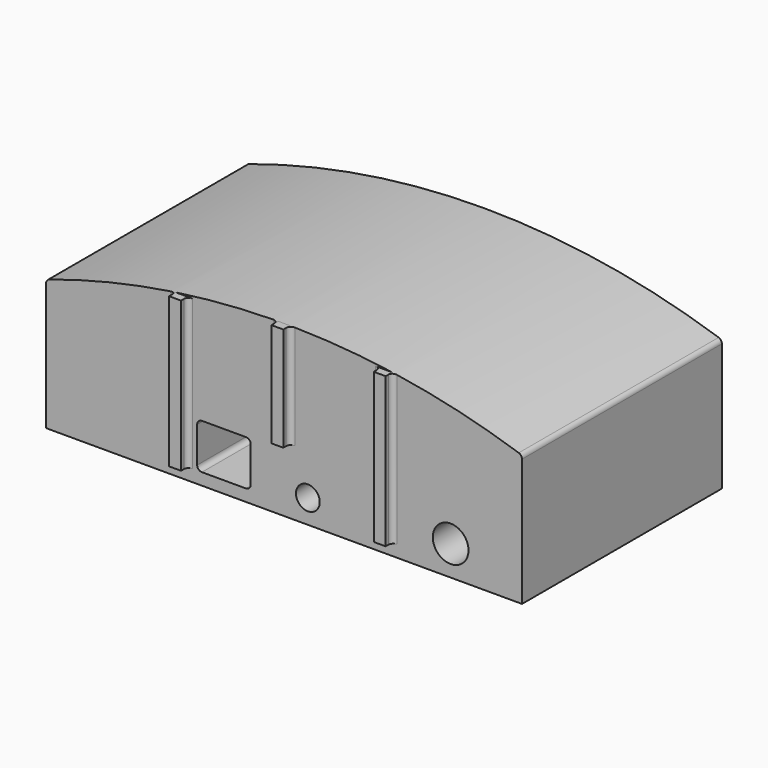
from build123d import *

# Parameters (mm, degrees)
F0_W         = 450
F0_H         = 380
F0_R         = 100
F0_R_2       = 150
F1_DEPTH     = 1050
F2_W         = 100
F2_H         = 1259.1041287501
F2_H_2       = 874.8020976761
F3_DEPTH     = 70
F4_T1_DEPTH  = 2100
F4_T3_DEPTH  = 1259.1041287501
F4_T8_DEPTH  = 1259.1041287501
F4_S9_R      = 6316.3461538462
F4_T10_DEPTH = 632
F4_T14_DEPTH = 874.8020976761
F4_S15_R     = 6316.3461538462
F4_T16_DEPTH = 440
F4_T20_DEPTH = 874.8020976761
F4_S21_R     = 6316.3461538462
F4_T22_DEPTH = 440
F4_T26_DEPTH = 1259.1041287501
F4_S27_R     = 6316.3461538462
F4_T28_DEPTH = 632
F4_T29_DEPTH = 2244.8937294243


# Not quite as in the source:
# - a fillet or chamfer that OpenCascade refuses, or shapes differently, is made with other operations: its cross-section is extruded or revolved along the edge and cut away or added


with BuildPart() as f1:
    # F0 (on Front) → F1 (new body, symmetric)
    with BuildSketch(Plane.XZ):
        with BuildLine():
            Line((-2000, -550), (2000, -550))
            Line((2000, -550), (2000, 550))
            ThreePointArc((2000, 550), (0, 875), (-2000, 550))
            Line((-2000, 550), (-2000, -550))
        make_face()
        with Locations((-505, -260)):
            Rectangle(F0_W, F0_H, mode=Mode.SUBTRACT)
        with Locations((200, -350)):
            Circle(F0_R, mode=Mode.SUBTRACT)
        with Locations((1400, -300)):
            Circle(F0_R_2, mode=Mode.SUBTRACT)
    extrude(amount=F1_DEPTH, both=True)

    # F2 (on face) → F3 (join)
    with BuildSketch(Plane.XZ.offset(1050)):
        with Locations((-860, 179.552064375)):
            Rectangle(F2_W, F2_H)
        with Locations((0, 437.401048838)):
            Rectangle(F2_W, F2_H_2)
        with Locations((860, 179.552064375)):
            Rectangle(F2_W, F2_H)
    extrude(amount=F3_DEPTH)

    # F4: fillet of radius 40 on 12 edges, made by hand

    # F4_s2 → F4_t1 (join)
    with BuildSketch(Plane.XZ.offset(-1050)):
        with BuildLine():
            ThreePointArc((-730, -410), (-718.2842712475, -438.2842712475), (-690, -450))
            Line((-690, -450), (-730, -450))
            Line((-730, -450), (-730, -410))
        make_face()
        with BuildLine():
            ThreePointArc((-730, -110), (-718.2842712475, -81.7157287525), (-690, -70))
            Line((-690, -70), (-730, -70))
            Line((-730, -70), (-730, -110))
        make_face()
        with BuildLine():
            ThreePointArc((-280, -410), (-291.7157287525, -438.2842712475), (-320, -450))
            Line((-320, -450), (-280, -450))
            Line((-280, -450), (-280, -410))
        make_face()
        with BuildLine():
            ThreePointArc((-320, -70), (-291.7157287525, -81.7157287525), (-280, -110))
            Line((-280, -110), (-280, -70))
            Line((-280, -70), (-320, -70))
        make_face()
    extrude(amount=F4_T1_DEPTH)

    # F4_s4 → F4_t3 (join)
    with BuildSketch(Plane.XY.offset(-450)):
        with BuildLine():
            ThreePointArc((-770, -1050), (-798.2842712475, -1061.7157287525), (-810, -1090))
            Line((-810, -1090), (-810, -1050))
            Line((-810, -1050), (-770, -1050))
        make_face()
        with BuildLine():
            ThreePointArc((770, -1050), (798.2842712475, -1061.7157287525), (810, -1090))
            Line((810, -1090), (810, -1050))
            Line((810, -1050), (770, -1050))
        make_face()
    extrude(amount=F4_T3_DEPTH)


with BuildPart() as f4_tool6:
    # F4_s7 → F4_t8 (new body)
    with BuildSketch(Plane.XY.offset(-450)):
        with BuildLine():
            ThreePointArc((950, -1050), (921.7157287525, -1061.7157287525), (910, -1090))
            Line((910, -1090), (910, -1050))
            Line((910, -1050), (950, -1050))
        make_face()
    extrude(amount=F4_T8_DEPTH)

    # F4_s9 → F4_t10 (intersect, symmetric)
    with BuildSketch(Plane.XZ.offset(1070)):
        with Locations((0, -5441.3461538462)):
            Circle(F4_S9_R)
    extrude(amount=F4_T10_DEPTH, both=True, mode=Mode.INTERSECT)


with BuildPart() as f1_1:
    add(f1.part)

    # F4_t5: union F4_tool6
    add(f4_tool6.part)


with BuildPart() as f4_tool12:
    # F4_s13 → F4_t14 (new body)
    with BuildSketch(Plane.XY):
        with BuildLine():
            ThreePointArc((90, -1050), (61.7157287525, -1061.7157287525), (50, -1090))
            Line((50, -1090), (50, -1050))
            Line((50, -1050), (90, -1050))
        make_face()
    extrude(amount=F4_T14_DEPTH)

    # F4_s15 → F4_t16 (intersect, symmetric)
    with BuildSketch(Plane.XZ.offset(1070)):
        with Locations((0, -5441.3461538462)):
            Circle(F4_S15_R)
    extrude(amount=F4_T16_DEPTH, both=True, mode=Mode.INTERSECT)


with BuildPart() as f1_2:
    add(f1_1.part)

    # F4_t11: union F4_tool12
    add(f4_tool12.part)


with BuildPart() as f4_tool18:
    # F4_s19 → F4_t20 (new body)
    with BuildSketch(Plane.XY.offset(874.8020976761)):
        with BuildLine():
            ThreePointArc((-90, -1050), (-61.7157287525, -1061.7157287525), (-50, -1090))
            Line((-50, -1090), (-50, -1050))
            Line((-50, -1050), (-90, -1050))
        make_face()
    extrude(amount=-F4_T20_DEPTH)

    # F4_s21 → F4_t22 (intersect, symmetric)
    with BuildSketch(Plane.XZ.offset(1070)):
        with Locations((0, -5441.3461538462)):
            Circle(F4_S21_R)
    extrude(amount=F4_T22_DEPTH, both=True, mode=Mode.INTERSECT)


with BuildPart() as f1_3:
    add(f1_2.part)

    # F4_t17: union F4_tool18
    add(f4_tool18.part)


with BuildPart() as f4_tool24:
    # F4_s25 → F4_t26 (new body)
    with BuildSketch(Plane.XY.offset(809.1041287501)):
        with BuildLine():
            ThreePointArc((-950, -1050), (-921.7157287525, -1061.7157287525), (-910, -1090))
            Line((-910, -1090), (-910, -1050))
            Line((-910, -1050), (-950, -1050))
        make_face()
    extrude(amount=-F4_T26_DEPTH)

    # F4_s27 → F4_t28 (intersect, symmetric)
    with BuildSketch(Plane.XZ.offset(1070)):
        with Locations((0, -5441.3461538462)):
            Circle(F4_S27_R)
    extrude(amount=F4_T28_DEPTH, both=True, mode=Mode.INTERSECT)


with BuildPart() as f1_4:
    add(f1_3.part)

    # F4_t23: union F4_tool24
    add(f4_tool24.part)

    # F4_s30 → F4_t29 (cut)
    with BuildSketch(Plane.XZ.offset(-1122.4468647121)):
        with BuildLine():
            ThreePointArc((1972.4913441799, 559.1127146357), (1992.4010321379, 544.5689271514), (2000, 521.1131577886))
            Line((2000, 521.1131577886), (2000, 550))
            ThreePointArc((2000, 550), (1986.2508981214, 554.5721331987), (1972.4913441799, 559.1127146357))
        make_face()
        with BuildLine():
            ThreePointArc((-2000, 521.1131577886), (-1992.4010321379, 544.5689271514), (-1972.4913441799, 559.1127146357))
            ThreePointArc((-1972.4913441799, 559.1127146357), (-1986.2508981214, 554.5721331987), (-2000, 550))
            Line((-2000, 550), (-2000, 521.1131577886))
        make_face()
    extrude(amount=F4_T29_DEPTH, mode=Mode.SUBTRACT)


solid = f1_4.part
